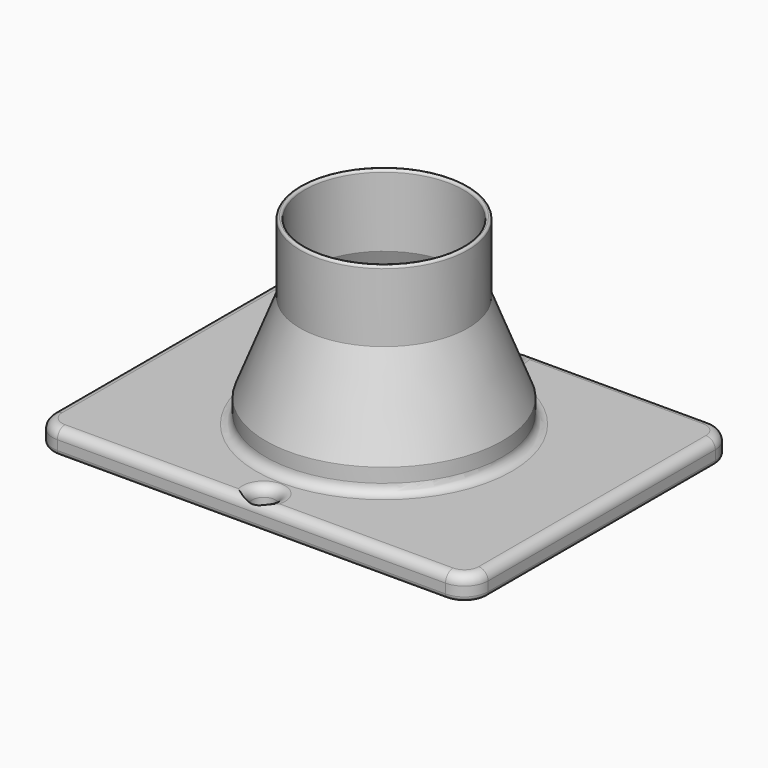
from build123d import *

# Parameters (mm, degrees)
F3_W          = 92
F3_H          = 70
F3_R          = 2.5
F4_DEPTH      = 5
F5_R          = 23.5
F6_DEPTH      = 5
F7_T3_DEPTH   = 102
F7_T5_DEPTH   = 80
F8_T1_DEPTH   = 17.4999999999
F8_T4_ANGLE   = 90
F8_T6_ANGLE   = 90
F8_T8_ANGLE   = 90
F8_T10_ANGLE  = 90
F9_R          = 0.49999
F10_T1_DEPTH  = 60
F10_T3_DEPTH  = 82
F10_T6_ANGLE  = 89.9999999974
F10_T8_ANGLE  = 89.9999999974
F10_T10_ANGLE = 89.9999999974
F10_T12_ANGLE = 89.9999999974


# Not quite as in the source:
# - a fillet or chamfer that OpenCascade refuses, or shapes differently, is made with other operations: its cross-section is extruded or revolved along the edge and cut away or added
# - a fillet or chamfer is up to 0.001 mm smaller than in the source, because OpenCascade refuses the exact size


with BuildPart() as f1:
    # F0 (on Front) → F1 (revolve)
    with BuildSketch(Plane.XZ):
        Polygon((-25, 10), (-25, 0), (-24, 0), (-24, 9.8123690243), (-16.75, 28.4520444507), (-16.75, 43.6396754264), (-17.75, 43.6396754264), (-17.75, 28.6396754264), align=None)
    revolve(axis=Axis((0, 0, 23.4480407089), (0, 0, 1)))

    # F3 (on offset) → F4 (join)
    with BuildSketch(Plane(origin=(0, 0, 0), x_dir=(1, 0, 0), z_dir=(0, 0, -1))):
        Rectangle(F3_W, F3_H)
        with Locations((0, -31.75)):
            Circle(F3_R, mode=Mode.SUBTRACT)
        with Locations((0, 31.75)):
            Circle(F3_R, mode=Mode.SUBTRACT)
    extrude(amount=-F4_DEPTH)

    # F5 (on face) → F6 (cut, through all)
    with BuildSketch(Plane(origin=(0, 0, 0), x_dir=(1, 0, 0), z_dir=(0, 0, -1))):
        Circle(F5_R)
    extrude(amount=-F6_DEPTH, mode=Mode.SUBTRACT)

    # F7: fillet of radius 2 on 7 edges, made by hand

    # F7_s1 → F7_t2 (revolve)
    with BuildSketch(Plane.XZ):
        with BuildLine():
            ThreePointArc((-25, 7), (-25.5857864376, 5.5857864376), (-27, 5))
            Line((-27, 5), (-25, 5))
            Line((-25, 5), (-25, 7))
        make_face()
    revolve(axis=Axis((0, 0, 5), (0, 0, -1)))

    # F7_s4 → F7_t3 (cut)
    with BuildSketch(Plane.YZ.offset(-51)):
        with BuildLine():
            ThreePointArc((-35, 3), (-34.4142135624, 4.4142135624), (-33, 5))
            Line((-33, 5), (-35, 5))
            Line((-35, 5), (-35, 3))
        make_face()
        with BuildLine():
            ThreePointArc((35, 3), (34.4142135624, 4.4142135624), (33, 5))
            Line((33, 5), (35, 5))
            Line((35, 5), (35, 3))
        make_face()
    extrude(amount=F7_T3_DEPTH, mode=Mode.SUBTRACT)

    # F7_s6 → F7_t5 (cut)
    with BuildSketch(Plane.XZ.offset(-40)):
        with BuildLine():
            ThreePointArc((46, 3), (45.4142135624, 4.4142135624), (44, 5))
            Line((44, 5), (46, 5))
            Line((46, 5), (46, 3))
        make_face()
        with BuildLine():
            ThreePointArc((-46, 3), (-45.4142135624, 4.4142135624), (-44, 5))
            Line((-44, 5), (-46, 5))
            Line((-46, 5), (-46, 3))
        make_face()
    extrude(amount=F7_T5_DEPTH, mode=Mode.SUBTRACT)

    # F7_s7 → F7_t8 (revolve, cut)
    with BuildSketch(Plane.XZ.offset(-31.75)):
        with BuildLine():
            ThreePointArc((2.5, 3), (3.0857864376, 4.4142135624), (4.5, 5))
            Line((4.5, 5), (2.5, 5))
            Line((2.5, 5), (2.5, 3))
        make_face()
    revolve(axis=Axis((0, 31.75, 5), (0, 0, -1)), mode=Mode.SUBTRACT)

    # F7_s9 → F7_t10 (revolve, cut)
    with BuildSketch(Plane.XZ.offset(31.75)):
        with BuildLine():
            ThreePointArc((2.5, 3), (3.0857864376, 4.4142135624), (4.5, 5))
            Line((4.5, 5), (2.5, 5))
            Line((2.5, 5), (2.5, 3))
        make_face()
    revolve(axis=Axis((0, -31.75, 5), (0, 0, -1)), mode=Mode.SUBTRACT)

    # F8: fillet of radius 5 on 4 edges, made by hand

    # F8_s2 → F8_t1 (cut)
    with BuildSketch(Plane.XY.offset(-12.5)):
        with BuildLine():
            ThreePointArc((41, -35), (44.5355339059, -33.5355339059), (46, -30))
            Line((46, -30), (46, -35))
            Line((46, -35), (41, -35))
        make_face()
        with BuildLine():
            ThreePointArc((-41, -35), (-44.5355339059, -33.5355339059), (-46, -30))
            Line((-46, -30), (-46, -35))
            Line((-46, -35), (-41, -35))
        make_face()
        with BuildLine():
            ThreePointArc((-46, 30), (-44.5355339059, 33.5355339059), (-41, 35))
            Line((-41, 35), (-46, 35))
            Line((-46, 35), (-46, 30))
        make_face()
        with BuildLine():
            ThreePointArc((46, 30), (44.5355339059, 33.5355339059), (41, 35))
            Line((41, 35), (46, 35))
            Line((46, 35), (46, 30))
        make_face()
    extrude(amount=F8_T1_DEPTH, mode=Mode.SUBTRACT)

    # F8_s3 → F8_t4 (revolve, cut)
    with BuildSketch(Plane.XZ.offset(-30)):
        with BuildLine():
            ThreePointArc((44.0000000001, 5), (45.4142135624, 4.4142135624), (46, 3.0000000001))
            Line((46, 3.0000000001), (46, 5))
            Line((46, 5), (44.0000000001, 5))
        make_face()
    revolve(axis=Axis((41, 30, 5), (0, 0, 1)), revolution_arc=F8_T4_ANGLE, mode=Mode.SUBTRACT)

    # F8_s5 → F8_t6 (revolve, cut)
    with BuildSketch(Plane.YZ.offset(-41)):
        with BuildLine():
            ThreePointArc((33.0000000001, 5), (34.4142135624, 4.4142135624), (35, 3.0000000001))
            Line((35, 3.0000000001), (35, 5))
            Line((35, 5), (33.0000000001, 5))
        make_face()
    revolve(axis=Axis((-41, 30, 5), (0, 0, 1)), revolution_arc=F8_T6_ANGLE, mode=Mode.SUBTRACT)

    # F8_s7 → F8_t8 (revolve, cut)
    with BuildSketch(Plane.XZ.offset(30)):
        with BuildLine():
            ThreePointArc((-44.0000000001, 5), (-45.4142135624, 4.4142135624), (-46, 3.0000000001))
            Line((-46, 3.0000000001), (-46, 5))
            Line((-46, 5), (-44.0000000001, 5))
        make_face()
    revolve(axis=Axis((-41, -30, 5), (0, 0, 1)), revolution_arc=F8_T8_ANGLE, mode=Mode.SUBTRACT)

    # F8_s9 → F8_t10 (revolve, cut)
    with BuildSketch(Plane.YZ.offset(41)):
        with BuildLine():
            ThreePointArc((-33.0000000001, 5), (-34.4142135624, 4.4142135624), (-35, 3.0000000001))
            Line((-35, 3.0000000001), (-35, 5))
            Line((-35, 5), (-33.0000000001, 5))
        make_face()
    revolve(axis=Axis((41, -30, 5), (0, 0, 1)), revolution_arc=F8_T10_ANGLE, mode=Mode.SUBTRACT)

    # F9 (radius 0.5 in the source; OpenCascade refuses exactly that, so slightly less here)
    f9_edges = [f1.edges().sort_by_distance(p)[0] for p in [
        (16.75, 0, 43.639675),
        (17.75, 0, 43.639675),
    ]]
    fillet(f9_edges, radius=F9_R)

    # F10: fillet of radius 1 on 11 edges, made by hand

    # F10_s2 → F10_t1 (cut)
    with BuildSketch(Plane.XZ.offset(-30)):
        with BuildLine():
            ThreePointArc((45, 0), (45.7071067812, 0.2928932188), (46, 1))
            Line((46, 1), (46, 0))
            Line((46, 0), (45, 0))
        make_face()
        with BuildLine():
            ThreePointArc((-45, 0), (-45.7071067812, 0.2928932188), (-46, 1))
            Line((-46, 1), (-46, 0))
            Line((-46, 0), (-45, 0))
        make_face()
    extrude(amount=F10_T1_DEPTH, mode=Mode.SUBTRACT)

    # F10_s4 → F10_t3 (cut)
    with BuildSketch(Plane.YZ.offset(-41)):
        with BuildLine():
            ThreePointArc((34, 0), (34.7071067812, 0.2928932188), (35, 1))
            Line((35, 1), (35, 0))
            Line((35, 0), (34, 0))
        make_face()
        with BuildLine():
            ThreePointArc((-34, 0), (-34.7071067812, 0.2928932188), (-35, 1))
            Line((-35, 1), (-35, 0))
            Line((-35, 0), (-34, 0))
        make_face()
    extrude(amount=F10_T3_DEPTH, mode=Mode.SUBTRACT)

    # F10_s5 → F10_t6 (revolve, cut)
    with BuildSketch(Plane.XZ.offset(29.9999999999)):
        with BuildLine():
            ThreePointArc((45, 0), (45.7071067812, 0.2928932188), (46, 1))
            Line((46, 1), (46, 0))
            Line((46, 0), (45, 0))
        make_face()
    revolve(axis=Axis((40.9999999999, -29.9999999999, 0), (0, 0, -1)), revolution_arc=F10_T6_ANGLE, mode=Mode.SUBTRACT)

    # F10_s7 → F10_t8 (revolve, cut)
    with BuildSketch(Plane.YZ.offset(40.9999999999)):
        with BuildLine():
            ThreePointArc((34, 0), (34.7071067812, 0.2928932188), (35, 1))
            Line((35, 1), (35, 0))
            Line((35, 0), (34, 0))
        make_face()
    revolve(axis=Axis((40.9999999999, 29.9999999999, 0), (0, 0, -1)), revolution_arc=F10_T8_ANGLE, mode=Mode.SUBTRACT)

    # F10_s9 → F10_t10 (revolve, cut)
    with BuildSketch(Plane.XZ.offset(-29.9999999999)):
        with BuildLine():
            ThreePointArc((-45, 0), (-45.7071067812, 0.2928932188), (-46, 1))
            Line((-46, 1), (-46, 0))
            Line((-46, 0), (-45, 0))
        make_face()
    revolve(axis=Axis((-40.9999999999, 29.9999999999, 0), (0, 0, -1)), revolution_arc=F10_T10_ANGLE, mode=Mode.SUBTRACT)

    # F10_s11 → F10_t12 (revolve, cut)
    with BuildSketch(Plane.YZ.offset(-40.9999999999)):
        with BuildLine():
            ThreePointArc((-34, 0), (-34.7071067812, 0.2928932188), (-35, 1))
            Line((-35, 1), (-35, 0))
            Line((-35, 0), (-34, 0))
        make_face()
    revolve(axis=Axis((-40.9999999999, -29.9999999999, 0), (0, 0, -1)), revolution_arc=F10_T12_ANGLE, mode=Mode.SUBTRACT)

    # F10_s13 → F10_t14 (revolve, cut)
    with BuildSketch(Plane.XZ.offset(-31.75)):
        with BuildLine():
            ThreePointArc((3.5, 0), (2.7928932188, 0.2928932188), (2.5, 1))
            Line((2.5, 1), (2.5, 0))
            Line((2.5, 0), (3.5, 0))
        make_face()
    revolve(axis=Axis((0, 31.75, 0), (0, 0, -1)), mode=Mode.SUBTRACT)

    # F10_s15 → F10_t16 (revolve, cut)
    with BuildSketch(Plane.XZ):
        with BuildLine():
            ThreePointArc((23.5, 1), (23.7928932188, 0.2928932188), (24.5, 0))
            Line((24.5, 0), (23.5, 0))
            Line((23.5, 0), (23.5, 1))
        make_face()
    revolve(axis=Axis((0, 0, 0), (0, 0, -1)), mode=Mode.SUBTRACT)

    # F10_s17 → F10_t18 (revolve, cut)
    with BuildSketch(Plane.XZ.offset(31.75)):
        with BuildLine():
            ThreePointArc((3.5, 0), (2.7928932188, 0.2928932188), (2.5, 1))
            Line((2.5, 1), (2.5, 0))
            Line((2.5, 0), (3.5, 0))
        make_face()
    revolve(axis=Axis((0, -31.75, 0), (0, 0, -1)), mode=Mode.SUBTRACT)


solid = f1.part
